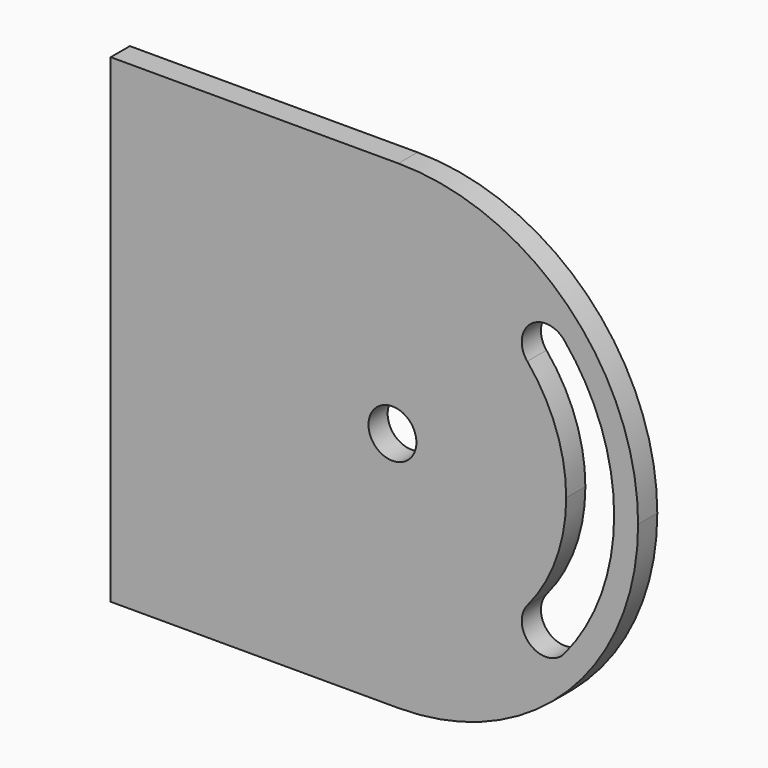
from build123d import *

# Parameters (mm, degrees)
F1_DEPTH = 3.175
F3_DEPTH = 3.175


# Not quite as in the source:
# - a feature names something its author has since deleted; it is built from what else it names


with BuildPart() as f1:
    # F0 (on Front) → F1 (new body)
    with BuildSketch(Plane.XZ):
        with BuildLine():
            Line((0, 63.5), (0, 0))
            Line((0, 0), (38.1, 0))
            ThreePointArc((38.1, 0), (60.5506403027, 9.2993596973), (69.85, 31.75))
            ThreePointArc((69.85, 31.75), (60.5506403027, 54.2006403027), (38.1, 63.5))
            Line((38.1, 63.5), (0, 63.5))
        make_face()
        with BuildLine():
            ThreePointArc((60.0519230645, 50.0432692204), (64.9682603323, 41.4776519117), (66.675, 31.75))
            ThreePointArc((66.675, 31.75), (64.9682603323, 22.0223480883), (60.0519230645, 13.4567307796))
            ThreePointArc((60.0519230645, 13.4567307796), (9.525, 31.75), (60.0519230645, 50.0432692204))
        make_face(mode=Mode.SUBTRACT)
        with BuildLine():
            ThreePointArc((55.1737179391, 17.5219017175), (58.997535814, 24.1840485131), (60.325, 31.75))
            ThreePointArc((60.325, 31.75), (58.997535814, 39.3159514869), (55.1737179391, 45.9780982825))
            ThreePointArc((55.1737179391, 45.9780982825), (15.875, 31.75), (55.1737179391, 17.5219017175))
        make_face()
        with BuildLine():
            ThreePointArc((55.1737179391, 45.9780982825), (55.5802350328, 50.4497863142), (60.0519230645, 50.0432692204))
            ThreePointArc((60.0519230645, 50.0432692204), (9.525, 31.75), (60.0519230645, 13.4567307796))
            ThreePointArc((60.0519230645, 13.4567307796), (55.5802350328, 13.0502136858), (55.1737179391, 17.5219017175))
            ThreePointArc((55.1737179391, 17.5219017175), (15.875, 31.75), (55.1737179391, 45.9780982825))
        make_face()
    extrude(amount=F1_DEPTH)

    # F2 (on face) → F3 (cut)
    with BuildSketch(Plane(origin=(0, 0, 0), x_dir=(-1, 0, 0), z_dir=(0, 1, 0))):
        with BuildLine():
            ThreePointArc((-34.1376, 31.75), (-37.3126, 34.925), (-40.4876, 31.75))
            ThreePointArc((-40.4876, 31.75), (-37.3126, 28.575), (-34.1376, 31.75))
        make_face()
    extrude(amount=-F3_DEPTH, mode=Mode.SUBTRACT)


solid = f1.part
